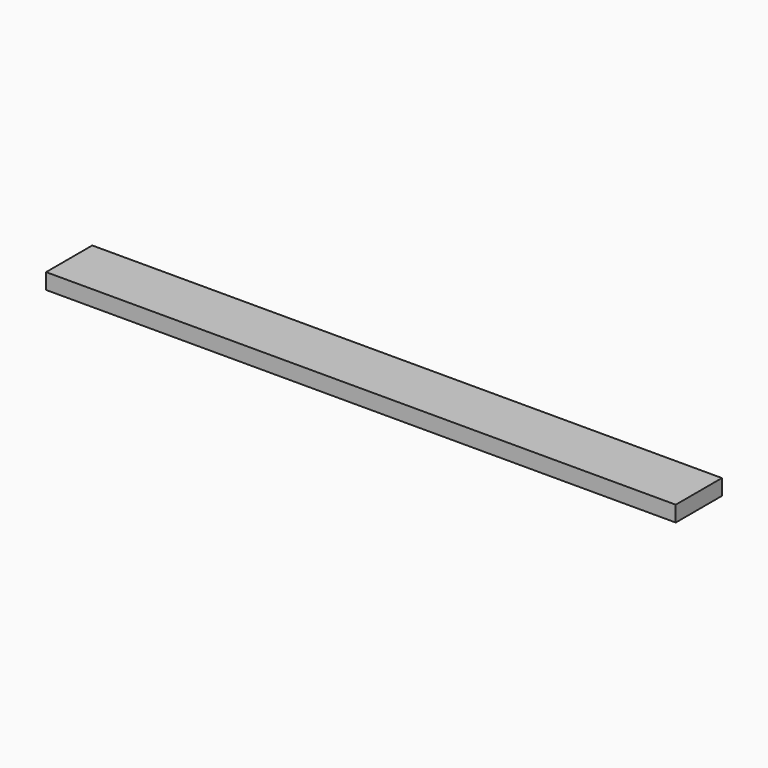
from build123d import *

# Parameters (mm, degrees)
F1_W     = 139.7
F1_H     = 38.1
F2_DEPTH = 762


# Not quite as in the source:
# - a variable given as a bare number and used for a length is read in inches; the dataset says mm whatever the document's units were


with BuildPart() as f2:
    # F1 (on Right) → F2 (new body, symmetric)
    with BuildSketch(Plane.YZ):
        Rectangle(F1_W, F1_H)
    extrude(amount=F2_DEPTH, both=True)


solid = f2.part
